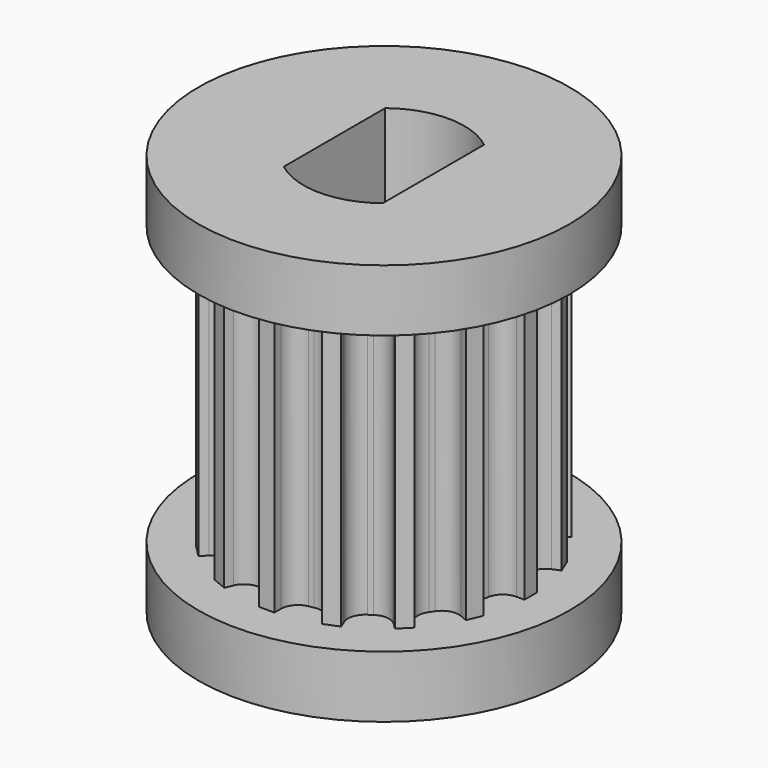
from build123d import *

# Parameters (mm, degrees)
F2_DEPTH        = 13
F1_R            = 6
F3_DEPTH        = 2
F4_DEPTH        = 13
F4_COPIES_COUNT = 16


# Not quite as in the source:
# - a pattern or mirror of a feature is missing from the dataset's text; its kind, count and spacing are read off the source's solid


with BuildPart() as f2:
    # F1 (on Top) → F2 (new body)
    with BuildSketch(Plane.XY):
        with BuildLine():
            ThreePointArc((-0.7033229276, -3.9389354049), (-0.4774392089, -3.9726473625), (-0.25, -3.9934164903))
            Line((-0.25, -3.9934164903), (0.25, -3.9934164903))
            Line((0.25, -3.9934164903), (0.7033229276, -3.9389354049))
            ThreePointArc((0.7033229276, -3.9389354049), (0, 4.0012342177), (-0.7033229276, -3.9389354049))
        make_face()
        with BuildLine():
            ThreePointArc((1.6, 2.0493901532), (2.3366642891, 1.1401754251), (2.6, 0))
            ThreePointArc((2.6, 0), (2.3366642891, -1.1401754251), (1.6, -2.0493901532))
            ThreePointArc((1.6, -2.0493901532), (0, -2.6), (-1.6, -2.0493901532))
            ThreePointArc((-1.6, -2.0493901532), (-2.6, 0), (-1.6, 2.0493901532))
            ThreePointArc((-1.6, 2.0493901532), (0, 2.6), (1.6, 2.0493901532))
        make_face(mode=Mode.SUBTRACT)
        with BuildLine():
            ThreePointArc((1.6, -2.0493901532), (2.3366642891, -1.1401754251), (2.6, 0))
            ThreePointArc((2.6, 0), (2.3366642891, 1.1401754251), (1.6, 2.0493901532))
            Line((1.6, 2.0493901532), (1.6, -2.0493901532))
        make_face()
        with BuildLine():
            Line((-1.6, -2.0493901532), (-1.6, 2.0493901532))
            ThreePointArc((-1.6, 2.0493901532), (-2.6, 0), (-1.6, -2.0493901532))
        make_face()
    extrude(amount=F2_DEPTH)

    # F1 (on Top) → F3 (join)
    with BuildSketch(Plane.XY):
        Circle(F1_R)
        with BuildLine():
            ThreePointArc((-0.25, -4.4803719605), (-0.3782937101, -4.1272943414), (-0.7033229276, -3.9389354049))
            ThreePointArc((-0.7033229276, -3.9389354049), (0, 4.0012342177), (0.7033229276, -3.9389354049))
            ThreePointArc((0.7033229276, -3.9389354049), (0.3782937101, -4.1272943414), (0.25, -4.4803719605))
            Line((0.25, -4.4803719605), (0.25, -4.7434164903))
            Line((0.25, -4.7434164903), (-0.25, -4.7434164903))
            Line((-0.25, -4.7434164903), (-0.25, -4.4803719605))
        make_face(mode=Mode.SUBTRACT)
    f3 = extrude(amount=F3_DEPTH)

    # F3_copies: F3 across plane
    add(f3.mirror(Plane.XY.offset(6.5)))

    # F1 (on Top) → F4 (join)
    with BuildSketch(Plane.XY):
        with BuildLine():
            Line((0.25, -3.9934164903), (-0.25, -3.9934164903))
            ThreePointArc((-0.25, -3.9934164903), (-0.4774392089, -3.9726473625), (-0.7033229276, -3.9389354049))
            ThreePointArc((-0.7033229276, -3.9389354049), (-0.3782937101, -4.1272943414), (-0.25, -4.4803719605))
            Line((-0.25, -4.4803719605), (-0.25, -4.7434164903))
            Line((-0.25, -4.7434164903), (0.25, -4.7434164903))
            Line((0.25, -4.7434164903), (0.25, -4.4803719605))
            ThreePointArc((0.25, -4.4803719605), (0.3782937101, -4.1272943414), (0.7033229276, -3.9389354049))
            Line((0.7033229276, -3.9389354049), (0.25, -3.9934164903))
        make_face()
    f4 = extrude(amount=F4_DEPTH)

    # F4_copies: F4 ×16 about axis
    f4_copies_axis = Axis((0, 0, 0), (0, 0, 1))
    for i in range(1, F4_COPIES_COUNT):
        add(f4.rotate(f4_copies_axis, i * 360 / F4_COPIES_COUNT))


solid = f2.part
